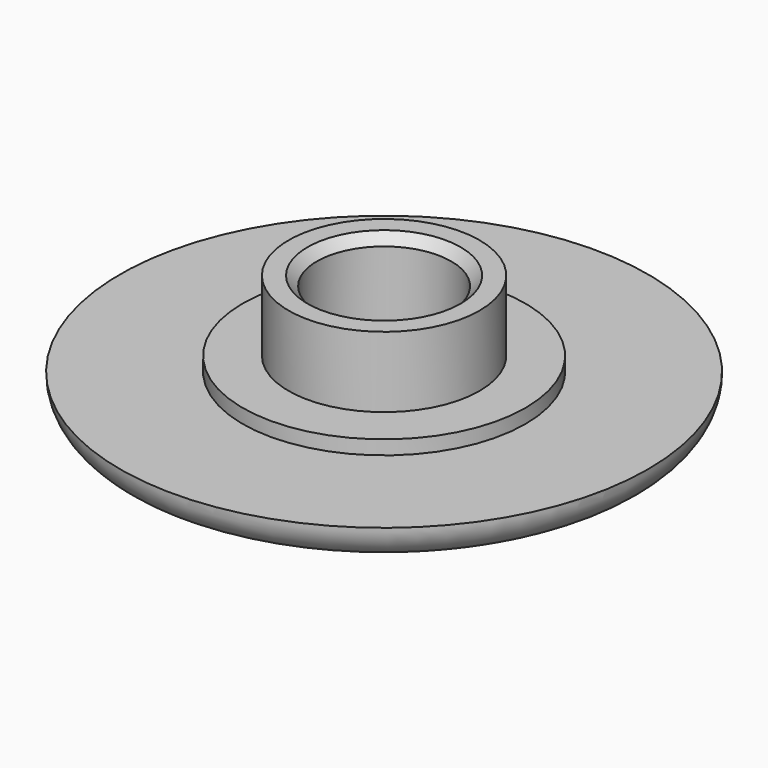
from build123d import *

# Parameters (mm, degrees)
F0_R     = 11.2
F1_DEPTH = 1.5
F2_R     = 6
F3_DEPTH = 0.6
F4_R     = 4.05
F5_DEPTH = 3
F6_T     = -1.2
F7_R     = 1.49999
F8_SIZE  = 0.4


# Not quite as in the source:
# - a fillet or chamfer is up to 0.001 mm smaller than in the source, because OpenCascade refuses the exact size


with BuildPart() as f1:
    # F0 (on Top) → F1 (new body)
    with BuildSketch(Plane.XY):
        Circle(F0_R)
    extrude(amount=-F1_DEPTH)

    # F2 (on face) → F3 (join)
    with BuildSketch(Plane.XY):
        Circle(F2_R)
    extrude(amount=F3_DEPTH)

    # F4 (on face) → F5 (join)
    with BuildSketch(Plane.XY.offset(0.6)):
        Circle(F4_R)
    extrude(amount=F5_DEPTH)

    # F6
    f6_openings = [f1.faces().sort_by_distance(p)[0] for p in [
        (0, 0, 3.6),
    ]]
    offset(amount=F6_T, openings=f6_openings, kind=Kind.INTERSECTION)

    # F7 (radius 1.5 in the source; OpenCascade refuses exactly that, so slightly less here)
    f7_edges = [f1.edges().sort_by_distance(p)[0] for p in [
        (-11.2, 0, -1.5),
    ]]
    fillet(f7_edges, radius=F7_R)

    # F8
    f8_edges = [f1.edges().sort_by_distance(p)[0] for p in [
        (-2.85, 0, 3.6),
        (2.85, 0, 1.65),
    ]]
    chamfer(f8_edges, length=F8_SIZE)


solid = f1.part
